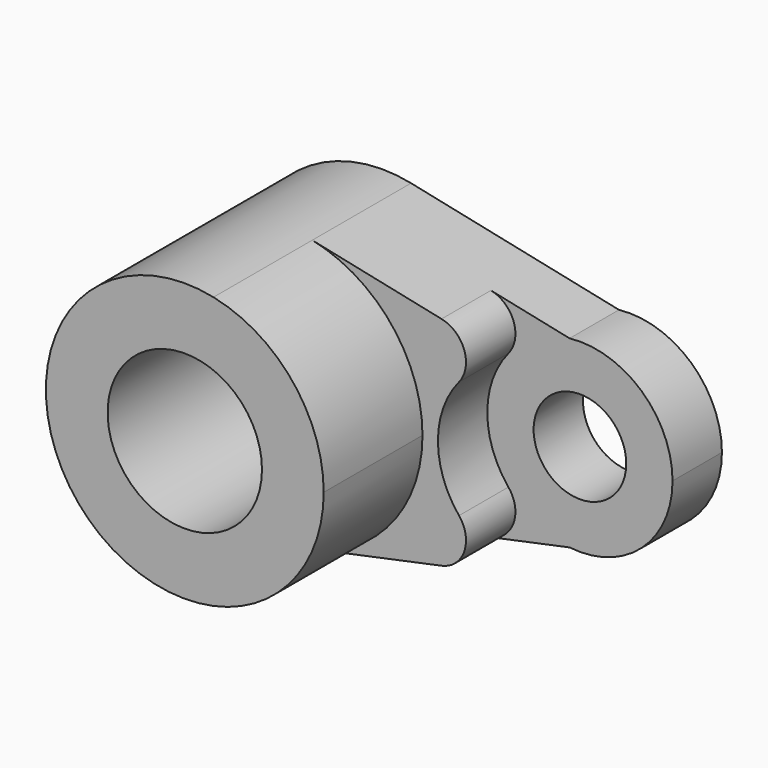
from build123d import *

# Parameters (mm, degrees)
F0_R     = 15.875
F0_R_2   = 9.525
F1_DEPTH = 25.4
F2_DEPTH = 25.4
F3_DEPTH = 12.7
F4_R     = 6.35


with BuildPart() as f1:
    # F0 (on Front) → F1 (new body)
    with BuildSketch(Plane.XZ):
        with BuildLine():
            ThreePointArc((5.9015777881, -27.9589342538), (22.1942358541, -17.998514379), (28.575, 0))
            ThreePointArc((28.575, 0), (22.1942358541, 17.998514379), (5.9015777881, 27.9589342538))
            ThreePointArc((5.9015777881, 27.9589342538), (-28.575, 0), (5.9015777881, -27.9589342538))
        make_face()
        Circle(F0_R, mode=Mode.SUBTRACT)
        with BuildLine():
            ThreePointArc((5.9015777881, 27.9589342538), (22.1942358541, 17.998514379), (28.575, 0))
            ThreePointArc((28.575, 0), (22.1942358541, -17.998514379), (5.9015777881, -27.9589342538))
            Line((5.9015777881, -27.9589342538), (48.6725341, -18.9308316998))
            ThreePointArc((48.6725341, -18.9308316998), (31.75, 0), (48.6725341, 18.9308316998))
            Line((48.6725341, 18.9308316998), (5.9015777881, 27.9589342538))
        make_face()
        with BuildLine():
            ThreePointArc((69.85, 0), (63.4959496416, 14.2026533682), (48.6725341, 18.9308316998))
            ThreePointArc((48.6725341, 18.9308316998), (31.75, 0), (48.6725341, -18.9308316998))
            ThreePointArc((48.6725341, -18.9308316998), (63.4959496416, -14.2026533682), (69.85, 0))
        make_face()
        with Locations((50.8, 0)):
            Circle(F0_R_2, mode=Mode.SUBTRACT)
    extrude(amount=-F1_DEPTH)

    # F0 (on Front) → F2 (join)
    with BuildSketch(Plane.XZ):
        with BuildLine():
            ThreePointArc((5.9015777881, -27.9589342538), (22.1942358541, -17.998514379), (28.575, 0))
            ThreePointArc((28.575, 0), (22.1942358541, 17.998514379), (5.9015777881, 27.9589342538))
            ThreePointArc((5.9015777881, 27.9589342538), (-28.575, 0), (5.9015777881, -27.9589342538))
        make_face()
        Circle(F0_R, mode=Mode.SUBTRACT)
    extrude(amount=F2_DEPTH)

    # F0 (on Front) → F3 (cut)
    with BuildSketch(Plane.XZ):
        with BuildLine():
            ThreePointArc((69.85, 0), (63.4959496416, 14.2026533682), (48.6725341, 18.9308316998))
            ThreePointArc((48.6725341, 18.9308316998), (31.75, 0), (48.6725341, -18.9308316998))
            ThreePointArc((48.6725341, -18.9308316998), (63.4959496416, -14.2026533682), (69.85, 0))
        make_face()
        with Locations((50.8, 0)):
            Circle(F0_R_2, mode=Mode.SUBTRACT)
    extrude(amount=-F3_DEPTH, mode=Mode.SUBTRACT)

    # F4
    f4_edges = [f1.edges().sort_by_distance(p)[0] for p in [
        (48.672534, 6.35, -18.930832),
        (48.672534, 6.35, 18.930832),
    ]]
    fillet(f4_edges, radius=F4_R)


solid = f1.part
